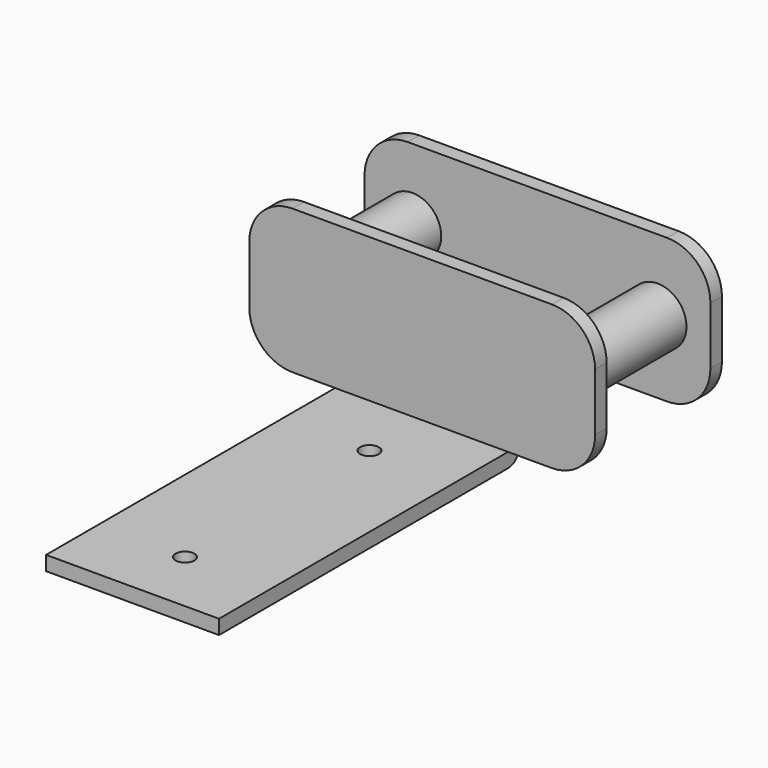
from build123d import *

# Parameters (mm, degrees)
F0_W     = 60
F0_H     = 130.3636354738
F1_DEPTH = 5
F3_DEPTH = 5
F4_R     = 10
F5_DEPTH = 50
F6_R     = 10
F7_DEPTH = 5
F9_D     = 6.5
F9_DEPTH = 6
F9_TIP   = 1.9527970118
F10_R    = 4.99999


# Not quite as in the source:
# - a fillet or chamfer is up to 0.001 mm smaller than in the source, because OpenCascade refuses the exact size


with BuildPart() as f1:
    # F0 (on Top) → F1 (new body)
    with BuildSketch(Plane.XY):
        with Locations((-0.2075759694, -49.6751572937)):
            Rectangle(F0_W, F0_H)
    extrude(amount=-F1_DEPTH)

    # F9
    with Locations(Plane(origin=(0, 0, -5), x_dir=(1, 0, 0), z_dir=(0, 0, -1))):
        with Locations((0, 12.3569750306), (0, 92.3569750306)):
            Hole(F9_D / 2, depth=F9_DEPTH)
            with Locations((0, 0, -(F9_DEPTH + F9_TIP / 2))):  # 118° drill point
                Cone(0, F9_D / 2, F9_TIP, mode=Mode.SUBTRACT)

    # F10 (radius 5 in the source; OpenCascade refuses exactly that, so slightly less here)
    f10_edges = [f1.edges().sort_by_distance(p)[0] for p in [
        (-0.207576, 15.50666, -5),
    ]]
    fillet(f10_edges, radius=F10_R)


with BuildPart() as f3:
    # F2 (on face) → F3 (new body)
    with BuildSketch(Plane(origin=(0, 15.5066604432, 0), x_dir=(-1, 0, 0), z_dir=(0, 1, 0))):
        with BuildLine():
            ThreePointArc((-60, 15), (-55.6066017178, 4.3933982822), (-45, 0))
            Line((-45, 0), (-29.7924240306, 0))
            Line((-29.7924240306, 0), (30.2075759694, 0))
            Line((30.2075759694, 0), (45, 0))
            ThreePointArc((45, 0), (55.6066017178, 4.3933982822), (60, 15))
            Line((60, 15), (60, 35))
            ThreePointArc((60, 35), (55.6066017178, 45.6066017178), (45, 50))
            Line((45, 50), (-45, 50))
            ThreePointArc((-45, 50), (-55.6066017178, 45.6066017178), (-60, 35))
            Line((-60, 35), (-60, 15))
        make_face()
    extrude(amount=-F3_DEPTH)

    # F4 (on face) → F5 (join)
    with BuildSketch(Plane(origin=(0, 15.5066604432, 0), x_dir=(-1, 0, 0), z_dir=(0, 1, 0))):
        with Locations((-41.705287993, 25)):
            Circle(F4_R)
        with Locations((43.3963425457, 25)):
            Circle(F4_R)
    extrude(amount=F5_DEPTH)

    # F6 (on face) → F7 (join)
    with BuildSketch(Plane(origin=(0, 65.5066604432, 0), x_dir=(-1, 0, 0), z_dir=(0, 1, 0))):
        with BuildLine():
            Line((-45, 0), (45, 0))
            ThreePointArc((45, 0), (55.6066017178, 4.3933982822), (60, 15))
            Line((60, 15), (60, 35))
            ThreePointArc((60, 35), (55.6066017178, 45.6066017178), (45, 50))
            Line((45, 50), (-45, 50))
            ThreePointArc((-45, 50), (-55.6066017178, 45.6066017178), (-60, 35))
            Line((-60, 35), (-60, 15))
            ThreePointArc((-60, 15), (-55.6066017178, 4.3933982822), (-45, 0))
        make_face()
        with Locations((-41.705287993, 25)):
            Circle(F6_R, mode=Mode.SUBTRACT)
    extrude(amount=-F7_DEPTH)


solid = Compound([f1.part, f3.part])
